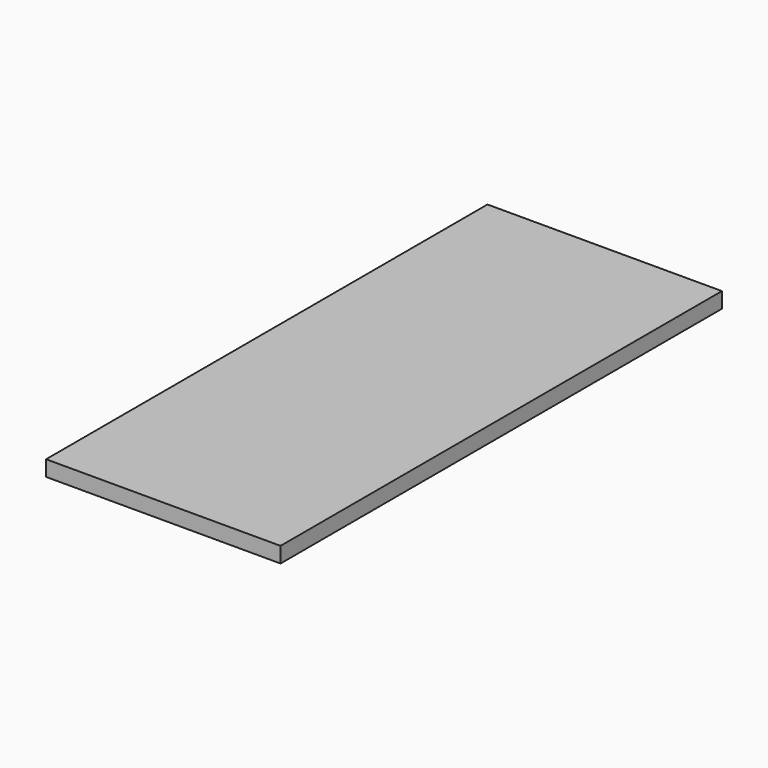
from build123d import *

# Parameters (mm, degrees)
F0_W     = 45.1724082232
F0_H     = 106.2966734171
F2_DEPTH = 3


# Not quite as in the source:
# - the program builds the solid bodies; features that only make, move or delete a surface that nothing else refers to are left out


with BuildPart() as f2:
    # F0 (on Top) → F2 (new body)
    with BuildSketch(Plane.XY):
        with Locations((22.5862041116, 53.1483367085)):
            Rectangle(F0_W, F0_H)
    extrude(amount=F2_DEPTH)


solid = f2.part
